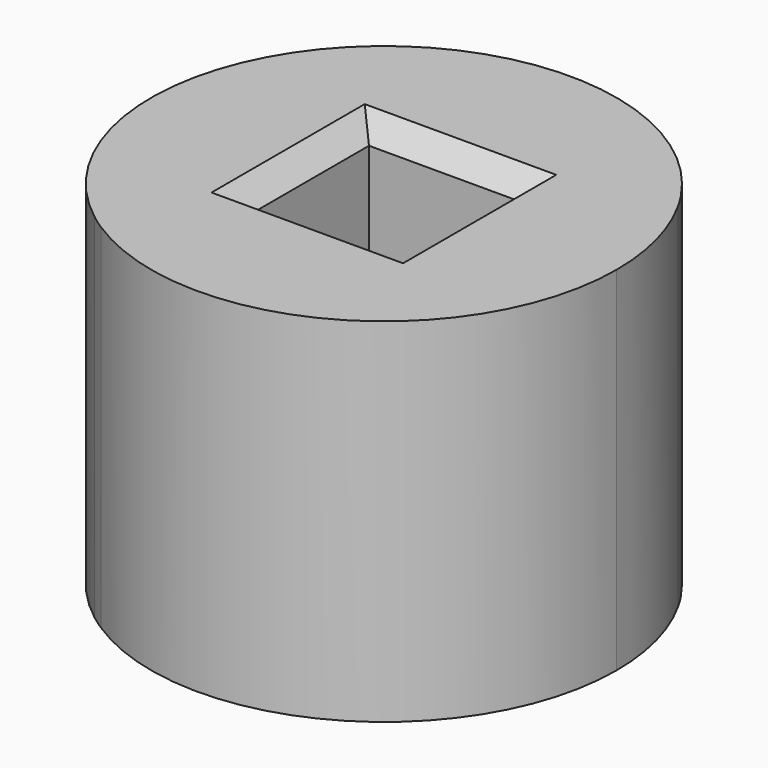
from build123d import *

# Parameters (mm, degrees)
F0_W     = 4.23
F0_H     = 4.23
F1_DEPTH = 10
F2_SIZE  = 0.6


# Not quite as in the source:
# - two fillets or chamfers of one size are made in one step


with BuildPart() as f1:
    # F0 (on Top) → F1 (new body)
    with BuildSketch(Plane.XY):
        with BuildLine():
            Line((-18.6, 10.6), (-9.2461221228, 10.6))
            ThreePointArc((-9.2461221228, 10.6), (-9.3644866857, 10.802164009), (-9.4899513299, 11))
            Line((-9.4899513299, 11), (-19, 11))
            Line((-19, 11), (-19, 2.1171452511))
            ThreePointArc((-19, 2.1171452511), (-18.8026143682, 1.9724540765), (-18.6, 1.8351804761))
            Line((-18.6, 1.8351804761), (-18.6, 10.6))
        make_face()
        with BuildLine():
            Line((-19, 11), (-9.4899513299, 11))
            ThreePointArc((-9.4899513299, 11), (-19.5051458211, 12.1901489162), (-19, 2.1171452511))
            Line((-19, 2.1171452511), (-19, 11))
        make_face()
        with BuildLine():
            ThreePointArc((-18.6, 1.8351804761), (-11.8535734555, 1.5651832687), (-8.4, 7.3669071504))
            ThreePointArc((-8.4, 7.3669071504), (-8.6150335165, 9.0378957815), (-9.2461221228, 10.6))
            Line((-9.2461221228, 10.6), (-18.6, 10.6))
            Line((-18.6, 10.6), (-18.6, 1.8351804761))
        make_face()
        with Locations((-15, 7.3669071504)):
            Rectangle(F0_W, F0_H, mode=Mode.SUBTRACT)
    extrude(amount=F1_DEPTH)

    # F2
    f2_edges = [f1.edges().sort_by_distance(p)[0] for p in [
        (-17.115, 7.366907, 10),
        (-15, 5.251907, 10),
        (-12.885, 7.366907, 10),
        (-15, 9.481907, 10),
        (-17.115, 7.366907, 0),
        (-15, 9.481907, 0),
        (-12.885, 7.366907, 0),
        (-15, 5.251907, 0),
    ]]
    chamfer(f2_edges, length=F2_SIZE)


solid = f1.part
